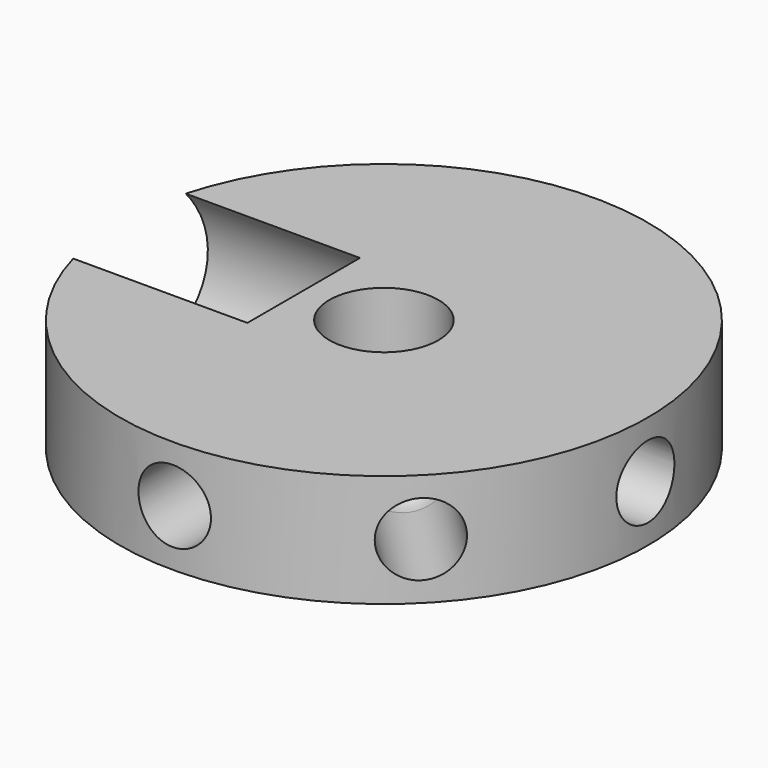
from build123d import *

# Parameters (mm, degrees)
F0_R             = 37.5
F1_DEPTH         = 16
F3_START         = -11.4
F2_R             = 12.8
F3_DEPTH         = 28.6
F4_R             = 7.75
F5_DEPTH         = 14
F12_COPIES_COUNT = 3
F12_COPIES_ANGLE = 90


# Not quite as in the source:
# - a pattern or mirror of a feature is missing from the dataset's text; its kind, count and spacing are read off the source's solid


with BuildPart() as f1:
    # F0 (on Top) → F1 (new body)
    with BuildSketch(Plane.XY):
        Circle(F0_R)
    extrude(amount=F1_DEPTH)

    # F2 (on Right) → F3 (cut)
    with BuildSketch(Plane.YZ.offset(F3_START)):
        with Locations((0, 8)):
            Circle(F2_R)
    extrude(amount=-F3_DEPTH, mode=Mode.SUBTRACT)

    # F4 (on face) → F5 (cut)
    with BuildSketch(Plane.XY.offset(16)):
        Circle(F4_R)
    extrude(amount=-F5_DEPTH, mode=Mode.SUBTRACT)

    # F7 (on Front) → F8 (revolve)
    with BuildSketch(Plane.XZ):
        Polygon((0, 2), (0, 4.4), (-2.2, 4.4), (-4.6, 2), align=None)
    revolve(axis=Axis((0, 0, 3.2), (0, 0, 1)))

    # F9 (on Front) → F10 (revolve, cut)
    with BuildSketch(Plane.XZ):
        with BuildLine():
            ThreePointArc((0, -10), (4.7376154339, -8.0376154339), (6.7, -3.3))
            ThreePointArc((6.7, -3.3), (4.7376154339, 1.4376154339), (0, 3.4))
            Line((0, 3.4), (0, -10))
        make_face()
    revolve(axis=Axis((0, 0, -3.3), (0, 0, -1)), mode=Mode.SUBTRACT)

    # F11 (on offset) → F12 (revolve, cut)
    with BuildSketch(Plane.XY.offset(8)):
        with BuildLine():
            Line((16, 0), (52, 0))
            Line((52, 0), (52, 5.15))
            Line((52, 5.15), (21.15, 5.15))
            ThreePointArc((21.15, 5.15), (17.5084000769, 3.6415999231), (16, 0))
        make_face()
    f12 = revolve(axis=Axis((34, 0, 8), (1, 0, 0)), mode=Mode.SUBTRACT)

    # F12_copies: F12 ×3 about axis
    f12_copies_axis = Axis((0, 0, 0), (0, 0, -1))
    for i in range(1, F12_COPIES_COUNT):
        add(f12.rotate(f12_copies_axis, i * F12_COPIES_ANGLE / (F12_COPIES_COUNT - 1)), mode=Mode.SUBTRACT)


solid = f1.part
